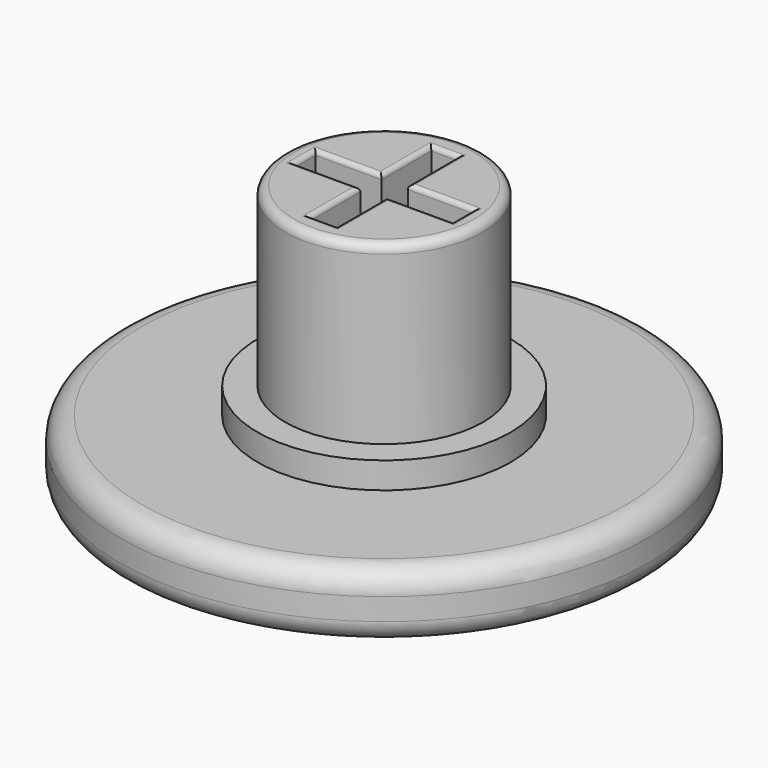
from build123d import *

# Parameters (mm, degrees)
F0_R      = 12
F1_DEPTH  = 3
F2_R      = 5.75
F3_DEPTH  = 1.2
F4_R      = 4.5
F5_DEPTH  = 8
F6_R      = 0.6
F10_DEPTH = 7
F11_W     = 1.2
F11_H     = 2.8315826069
F11_H_2   = 1.2
F11_W_2   = 2.9928033758
F12_DEPTH = 4
F13_R     = 0.4
F14_R     = 1
F15_R     = 0.2


# Not quite as in the source:
# - a feature of the source that left no trace in its solid (it failed there, or was rolled back) is left out


with BuildPart() as f1:
    # F0 (on Top) → F1 (new body)
    with BuildSketch(Plane.XY):
        Circle(F0_R)
    extrude(amount=F1_DEPTH)

    # F2 (on face) → F3 (join)
    with BuildSketch(Plane.XY.offset(3)):
        Circle(F2_R)
    extrude(amount=F3_DEPTH)

    # F4 (on face) → F5 (join)
    with BuildSketch(Plane.XY.offset(4.2)):
        Circle(F4_R)
    extrude(amount=F5_DEPTH)

    # F6 (on face) → F10 (cut)
    with BuildSketch(Plane.XY.offset(12.2)):
        Circle(F6_R)
    extrude(amount=-F10_DEPTH, mode=Mode.SUBTRACT)

    # F11 (on face) → F12 (cut)
    with BuildSketch(Plane.XY.offset(12.2)):
        with Locations((0, 2.0157913034)):
            Rectangle(F11_W, F11_H)
        Rectangle(F11_W, F11_H_2)
        with Locations((-2.0964016879, 0)):
            Rectangle(F11_W_2, F11_H_2)
        with Locations((2.0964016879, 0)):
            Rectangle(F11_W_2, F11_H_2)
        with Locations((0, -2.0157913034)):
            Rectangle(F11_W, F11_H)
    extrude(amount=-F12_DEPTH, mode=Mode.SUBTRACT)

    # F13
    f13_edges = [f1.edges().sort_by_distance(p)[0] for p in [
        (-4.5, 0, 12.2),
    ]]
    fillet(f13_edges, radius=F13_R)

    # F14
    f14_edges = [f1.edges().sort_by_distance(p)[0] for p in [
        (-12, 0, 3),
        (-12, 0, 0),
    ]]
    fillet(f14_edges, radius=F14_R)

    # F15
    f15_edges = [f1.edges().sort_by_distance(p)[0] for p in [
        (-4.1, 0, 12.2),
        (0, 3.431583, 12.2),
        (-0.6, 2.015791, 12.2),
        (-2.096402, 0.6, 12.2),
        (-3.592803, 0, 12.2),
        (-2.096402, -0.6, 12.2),
        (-0.6, -2.015791, 12.2),
        (0, -3.431583, 12.2),
        (0.6, -2.015791, 12.2),
        (2.096402, -0.6, 12.2),
        (3.592803, 0, 12.2),
        (2.096402, 0.6, 12.2),
        (0.6, 2.015791, 12.2),
        (-0.6, 0, 8.2),
    ]]
    fillet(f15_edges, radius=F15_R)


solid = f1.part
